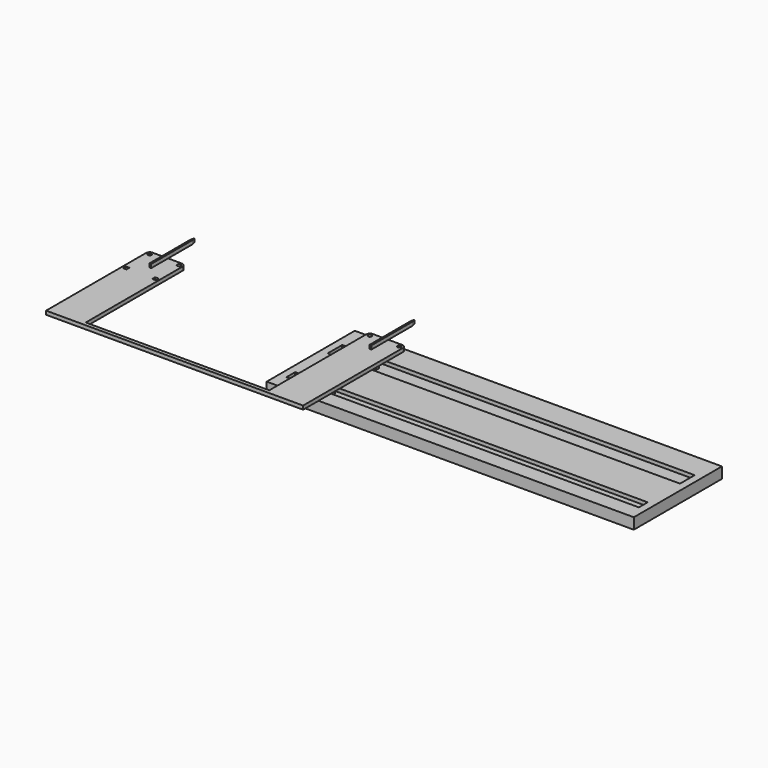
from build123d import *

# Parameters (mm, degrees)
F0_W      = 1
F0_H      = 1
F0_R      = 0.5
F0_W_2    = 50
F0_H_2    = 4.5
F1_DEPTH  = 1
F2_W      = 0.4784071445
F2_H      = 14
F3_DEPTH  = 1
F5_START  = -1
F4_W      = 100
F4_H      = 30
F4_W_2    = 96
F4_H_2    = 3
F4_H_3    = 5
F5_DEPTH  = 3
F6_DEPTH  = 25
F7_DEPTH  = 2
F8_DEPTH  = 2
F9_W      = 50
F9_H      = 28.5
F10_DEPTH = 25


with BuildPart() as f1:
    # F0 (on Top) → F1 (new body)
    with BuildSketch(Plane.XY):
        with BuildLine():
            Line((4.1333548725, -26.0610329807), (4.1333548725, -30.5610329807))
            Line((4.1333548725, -30.5610329807), (14.1333548725, -30.5610329807))
            Line((14.1333548725, -30.5610329807), (14.1333548725, -21.5610329807))
            ThreePointArc((14.1333548725, -21.5610329807), (13.8404616537, -20.8539261995), (13.1333548725, -20.5610329807))
            Line((13.1333548725, -20.5610329807), (5.1333548725, -20.5610329807))
            ThreePointArc((5.1333548725, -20.5610329807), (4.4262480913, -20.8539261995), (4.1333548725, -21.5610329807))
            Line((4.1333548725, -21.5610329807), (4.1333548725, -26.0610329807))
        make_face()
        with Locations((5.1333548725, -29.5610329807)):
            Rectangle(F0_W, F0_H, mode=Mode.SUBTRACT)
        with Locations((13.1333548725, -29.5610329807)):
            Rectangle(F0_W, F0_H, mode=Mode.SUBTRACT)
        with Locations((5.1333548725, -21.5610329807)):
            Circle(F0_R, mode=Mode.SUBTRACT)
        with Locations((13.1333548725, -21.5610329807)):
            Circle(F0_R, mode=Mode.SUBTRACT)
        with BuildLine():
            Line((-55.8666451275, -30.5610329807), (-45.8666451275, -30.5610329807))
            Line((-45.8666451275, -30.5610329807), (-45.8666451275, -26.0610329807))
            Line((-45.8666451275, -26.0610329807), (-45.8666451275, -21.5610329807))
            ThreePointArc((-45.8666451275, -21.5610329807), (-46.1595383463, -20.8539261995), (-46.8666451275, -20.5610329807))
            Line((-46.8666451275, -20.5610329807), (-54.8666451275, -20.5610329807))
            ThreePointArc((-54.8666451275, -20.5610329807), (-55.5737519087, -20.8539261995), (-55.8666451275, -21.5610329807))
            Line((-55.8666451275, -21.5610329807), (-55.8666451275, -30.5610329807))
        make_face()
        with Locations((-54.8666451275, -29.5610329807)):
            Rectangle(F0_W, F0_H, mode=Mode.SUBTRACT)
        with Locations((-46.8666451275, -29.5610329807)):
            Rectangle(F0_W, F0_H, mode=Mode.SUBTRACT)
        with Locations((-54.8666451275, -21.5610329807)):
            Circle(F0_R, mode=Mode.SUBTRACT)
        with Locations((-46.8666451275, -21.5610329807)):
            Circle(F0_R, mode=Mode.SUBTRACT)
        with Locations((-20.8666451275, -28.3110329807)):
            Rectangle(F0_W_2, F0_H_2)
    extrude(amount=-F1_DEPTH)

    # F6 (add): a face of the model
    f6_faces = [f1.faces().sort_by_distance(p)[0] for p in [
        (-20.8666451275, -30.5610329807, -0.5),
    ]]
    extrude(f6_faces, amount=F6_DEPTH)

    # F0 (on Top) → F8 (join, through all)
    with BuildSketch(Plane.XY):
        with Locations((13.1333548725, -44.5610329807)):
            Rectangle(F0_W, F0_H)
        with Locations((5.1333548725, -44.5610329807)):
            Rectangle(F0_W, F0_H)
        with Locations((5.1333548725, -29.5610329807)):
            Rectangle(F0_W, F0_H)
        with Locations((13.1333548725, -29.5610329807)):
            Rectangle(F0_W, F0_H)
    extrude(amount=-F8_DEPTH)

    # F9 (on face) → F10 (cut)
    with BuildSketch(Plane.XY):
        with Locations((-20.8666451275, -40.3110329807)):
            Rectangle(F9_W, F9_H)
    extrude(amount=-F10_DEPTH, mode=Mode.SUBTRACT)


with BuildPart() as f3:
    # F2 (on face) → F3 (new body)
    with BuildSketch(Plane.XY):
        Polygon((9.3725584447, -12.3256136095), (9.1333548725, -11.3256136095), (8.8941513002, -12.3256136095), align=None)
        with Locations((9.1333548725, -19.3256136095)):
            Rectangle(F2_W, F2_H)
    extrude(amount=F3_DEPTH)


with BuildPart() as f3b:
    # F2 (on face) → F3, piece 2 (new body)
    with BuildSketch(Plane.XY):
        Polygon((-51.1058486998, -12.3256136095), (-50.6274415553, -12.3256136095), (-50.8666451275, -11.3256136095), align=None)
        with Locations((-50.8666451275, -19.3256136095)):
            Rectangle(F2_W, F2_H)
    extrude(amount=F3_DEPTH)


with BuildPart() as f5:
    # F4 (on Top) → F5 (new body)
    with BuildSketch(Plane.XY.offset(F5_START)):
        with Locations((50, -35.2865339816)):
            Rectangle(F4_W, F4_H)
        with Locations((50, -44.5610329807)):
            Rectangle(F4_W_2, F4_H_2, mode=Mode.SUBTRACT)
        with Locations((50, -29.5610329807)):
            Rectangle(F4_W_2, F4_H_3, mode=Mode.SUBTRACT)
        with Locations((50, -44.5610329807)):
            Rectangle(F4_W_2, F4_H_2)
        with Locations((50, -29.5610329807)):
            Rectangle(F4_W_2, F4_H_3)
    extrude(amount=-F5_DEPTH)

    # F4 (on Top) → F7 (cut)
    with BuildSketch(Plane.XY):
        with Locations((50, -29.5610329807)):
            Rectangle(F4_W_2, F4_H_3)
        with Locations((50, -44.5610329807)):
            Rectangle(F4_W_2, F4_H_2)
    extrude(amount=-F7_DEPTH, mode=Mode.SUBTRACT)


solid = Compound([f1.part, f3.part, f3b.part, f5.part])
